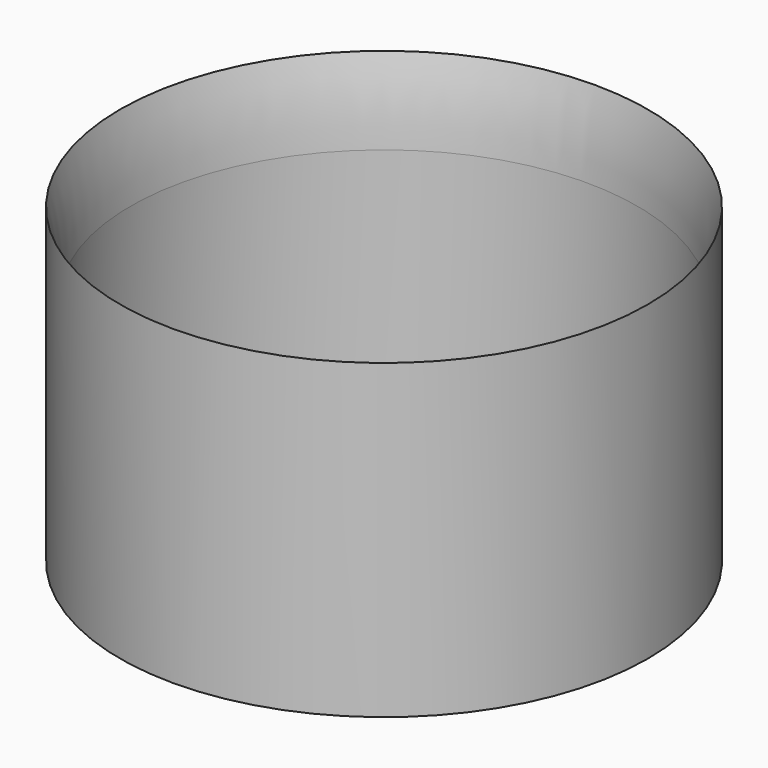
from build123d import *

# Parameters (mm, degrees)
F0_R     = 18.923
F0_R_2   = 18.161
F1_DEPTH = 22.352
F2_R     = 18.8764388906
F3_DEPTH = 1.27


# Not quite as in the source:
# - a fillet or chamfer that OpenCascade refuses, or shapes differently, is made with other operations: its cross-section is extruded or revolved along the edge and cut away or added


with BuildPart() as f1:
    # F0 (on Top) → F1 (new body)
    with BuildSketch(Plane.XY):
        Circle(F0_R)
        Circle(F0_R_2, mode=Mode.SUBTRACT)
    extrude(amount=F1_DEPTH)

    # F2 (on Top) → F3 (join)
    with BuildSketch(Plane.XY):
        Circle(F2_R)
    extrude(amount=F3_DEPTH)

    # F4: fillet of radius 22.86 on 1 edges, made by hand

    # F4_s1 → F4_t2 (revolve, cut)
    with BuildSketch(Plane.XZ):
        with BuildLine():
            ThreePointArc((18.923, 22.352), (18.3523004343, 19.4501802499), (18.161, 16.4989669401))
            Line((18.161, 16.4989669401), (18.161, 22.352))
            Line((18.161, 22.352), (18.923, 22.352))
        make_face()
    revolve(axis=Axis((0, 0, 22.352), (0, 0, 1)), mode=Mode.SUBTRACT)


solid = f1.part
